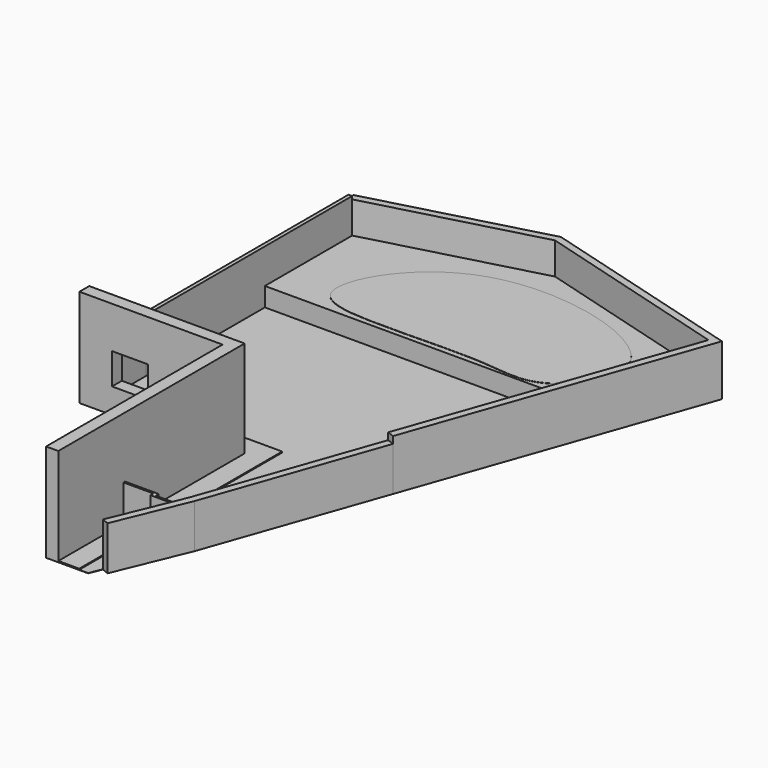
from build123d import *

# Parameters (mm, degrees)
F1_DEPTH  = 78
F2_DEPTH  = 5
F0_W      = 85
F0_H      = 332
F3_DEPTH  = 220
F4_DEPTH  = 220
F5_DEPTH  = 400
F6_W      = 167
F6_H      = 200
F6_W_2    = 146
F6_H_2    = 127
F7_DEPTH  = 200
F8_DEPTH  = 208
F9_DEPTH  = 180
F0_H_2    = 8
F0_W_2    = 37
F10_DEPTH = 152
F11_DEPTH = 79
F12_DEPTH = 1
F13_DEPTH = 1


# Not quite as in the source:
# - a feature names something its author has since deleted; it is built from what else it names


with BuildPart() as f1:
    # F0 (on Top) → F1 (new body)
    with BuildSketch(Plane.XY):
        Polygon((-741.2445402145, 1082.0436550353), (-741.2445402145, 636.6001187265), (85.7554597855, 636.6001187265), (611.9789830182, 636.6001187265), (751.3498777895, 1033.1027120147), (-59.6568852941, 1264.6745167422), align=None)
        with BuildLine():
            add(Edge.make_bspline(
                [(-333.5347517591, 657.5935368718), (-438.7176092773, 660.9860382691), (-660.4423976157, 691.4819966509), (-306.0983067038, 1304.6981771282), (678.1962489209, 1041.8383423681), (388.5420616008, 608.4940348272), (127.1086766673, 676.0293060865), (-184.2398763148, 652.7782743329), (-333.5347517591, 657.5935368718)],
                knots=[0, 0, 0, 0, 0.1269070803, 0.3114768491, 0.5429923215, 0.687036639, 0.8198701082, 1, 1, 1, 1], degree=3))
        make_face(mode=Mode.SUBTRACT)
    extrude(amount=F1_DEPTH)


with BuildPart() as f2:
    # F0 (on Top) → F2 (new body)
    with BuildSketch(Plane.XY):
        Polygon((-157.2445402145, -196.4231370871), (-157.2445402145, -333.8946764966), (-157.2445402145, -806.4231370871), (-72.2445402145, -806.4231370871), (-72.2445402145, -360.4946641021), (-72.2445402145, -111.4231370871), (-741.2445402145, -111.4231370871), (-741.2445402145, -196.4231370871), align=None)
    extrude(amount=F2_DEPTH)

    # F0 (on Top) → F3 (join)
    with BuildSketch(Plane.XY):
        Polygon((-791.2445402145, -196.4231370871), (-741.2445402145, -196.4231370871), (-741.2445402145, -111.4231370871), (-741.2445402145, 29.6001187267), (-756.2445402145, 29.6001187267), (-791.2445402145, 29.6001187267), align=None)
    extrude(amount=F3_DEPTH)

    # F0 (on Top) → F5 (join)
    with BuildSketch(Plane.XY):
        Polygon((-157.2445402145, -806.4231370871), (-157.2445402145, -333.8946764966), (-157.2445402145, -196.4231370871), (-741.2445402145, -196.4231370871), (-791.2445402145, -196.4231370871), (-791.2445402145, -246.4231370871), (-207.2444250903, -246.4231370871), (-207.2444250903, -1146.5304329774), (-157.2445402145, -1146.4231370871), (-157.2445402145, -814.4231370871), align=None)
    extrude(amount=F5_DEPTH)

    # F6 (on face) → F7 (cut)
    with BuildSketch(Plane(origin=(0, -196.4231370871, 0), x_dir=(-1, 0, 0), z_dir=(0, 1, 0))):
        with Locations((324.7445402145, 105)):
            Rectangle(F6_W, F6_H)
        with Locations((585.2445402145, 166.5)):
            Rectangle(F6_W_2, F6_H_2)
    extrude(amount=-F7_DEPTH, mode=Mode.SUBTRACT)


with BuildPart() as f2b:
    # F0 (on Top) → F2, piece 2 (new body)
    with BuildSketch(Plane.XY):
        with Locations((-114.7445402145, -980.4231370871)):
            Rectangle(F0_W, F0_H)
    extrude(amount=F2_DEPTH)


with BuildPart() as f4:
    # F0 (on Top) → F4 (new body)
    with BuildSketch(Plane.XY):
        Polygon((-756.2445402145, 29.6001187267), (-741.2445402145, 29.6001187267), (-741.2445402145, 636.6001187265), (-741.2445402145, 1082.0436550353), (-756.2445402145, 1082.0436550353), align=None)
    extrude(amount=F4_DEPTH)


with BuildPart() as f8:
    # F0 (on Top) → F8 (new body)
    with BuildSketch(Plane.XY):
        Polygon((-756.2445402145, 1082.0436550353), (-741.2445402145, 1082.0436550353), (-59.6568852941, 1264.6745167422), (751.3498777895, 1033.1027120147), (611.9789830182, 636.6001187265), (536.7554597855, 422.5932983858), (352.412635156, -101.8519822417), (380.7150506744, -111.8002979444), (790.2292767004, 1053.2451157589), (-59.6568852941, 1294.6745167422), (-756.2445402145, 1108.0244171488), align=None)
    extrude(amount=F8_DEPTH)


with BuildPart() as f9:
    # F0 (on Top) → F9 (new body)
    with BuildSketch(Plane.XY):
        Polygon((95.2382184061, -829.4231370871), (-15.2445402145, -1096.4231370871), (12.4759647581, -1107.8936908689), (133.0854861388, -816.292767618), (380.7150506744, -111.8002979444), (352.412635156, -101.8519822417), (104.7554597855, -806.4231370871), align=None)
    extrude(amount=F9_DEPTH)


with BuildPart() as f10:
    # F0 (on Top) → F10 (new body)
    with BuildSketch(Plane.XY):
        with Locations((-114.7445402145, -810.4231370871)):
            Rectangle(F0_W, F0_H_2)
        with Locations((-53.7445402145, -810.4231370871)):
            Rectangle(F0_W_2, F0_H_2)
        Polygon((-20.2445402145, -821.4231370871), (-35.2445402145, -821.4231370871), (-35.2445402145, -829.4231370871), (95.2382184061, -829.4231370871), (95.2382184061, -821.4231370871), align=None)
        Polygon((-20.2445402145, -806.4231370871), (-35.2445402145, -806.4231370871), (-35.2445402145, -814.4231370871), (-35.2445402145, -821.4231370871), (-20.2445402145, -821.4231370871), align=None)
    extrude(amount=F10_DEPTH)


with BuildPart() as f11:
    # F0 (on Top) → F11 (new body)
    with BuildSketch(Plane.XY):
        with BuildLine():
            add(Edge.make_bspline(
                [(-333.5347517591, 657.5935368718), (-438.7176092773, 660.9860382691), (-660.4423976157, 691.4819966509), (-306.0983067038, 1304.6981771282), (678.1962489209, 1041.8383423681), (388.5420616008, 608.4940348272), (127.1086766673, 676.0293060865), (-184.2398763148, 652.7782743329), (-333.5347517591, 657.5935368718)],
                knots=[0, 0, 0, 0, 0.1269070803, 0.3114768491, 0.5429923215, 0.687036639, 0.8198701082, 1, 1, 1, 1], degree=3))
        make_face()
    extrude(amount=F11_DEPTH)


with BuildPart() as f12:
    # F0 (on Top) → F12 (new body)
    with BuildSketch(Plane.XY):
        Polygon((-72.2445402145, -360.4946641021), (-72.2445402145, -806.4231370871), (-35.2445402145, -806.4231370871), (-20.2445402145, -806.4231370871), (-20.2445402145, -821.4231370871), (95.2382184061, -821.4231370871), (95.2382184061, -829.4231370871), (104.7554597855, -806.4231370871), (352.412635156, -101.8519822417), (536.7554597855, 422.5932983858), (430.7554597855, 422.5932983858), (310.7554597855, 422.5932983858), (85.7554597855, 422.5932983858), (85.7554597855, 636.6001187265), (-741.2445402145, 636.6001187265), (-741.2445402145, 29.6001187267), (-741.2445402145, -111.4231370871), (-72.2445402145, -111.4231370871), align=None)
        Polygon((611.9789830182, 636.6001187265), (85.7554597855, 636.6001187265), (85.7554597855, 422.5932983858), (310.7554597855, 422.5932983858), (430.7554597855, 422.5932983858), (536.7554597855, 422.5932983858), align=None)
    extrude(amount=F12_DEPTH)


with BuildPart() as f13:
    # F0 (on Top) → F13 (new body)
    with BuildSketch(Plane.XY):
        Polygon((-35.2445402145, -814.4231370871), (-72.2445402145, -814.4231370871), (-72.2445402145, -1146.4231370871), (-35.934195387, -1146.4231370871), (-15.2445402145, -1096.4231370871), (95.2382184061, -829.4231370871), (-35.2445402145, -829.4231370871), (-35.2445402145, -821.4231370871), align=None)
    extrude(amount=F13_DEPTH)


solid = Compound([f1.part, f2.part, f2b.part, f4.part, f8.part, f9.part, f10.part, f11.part, f12.part, f13.part])
